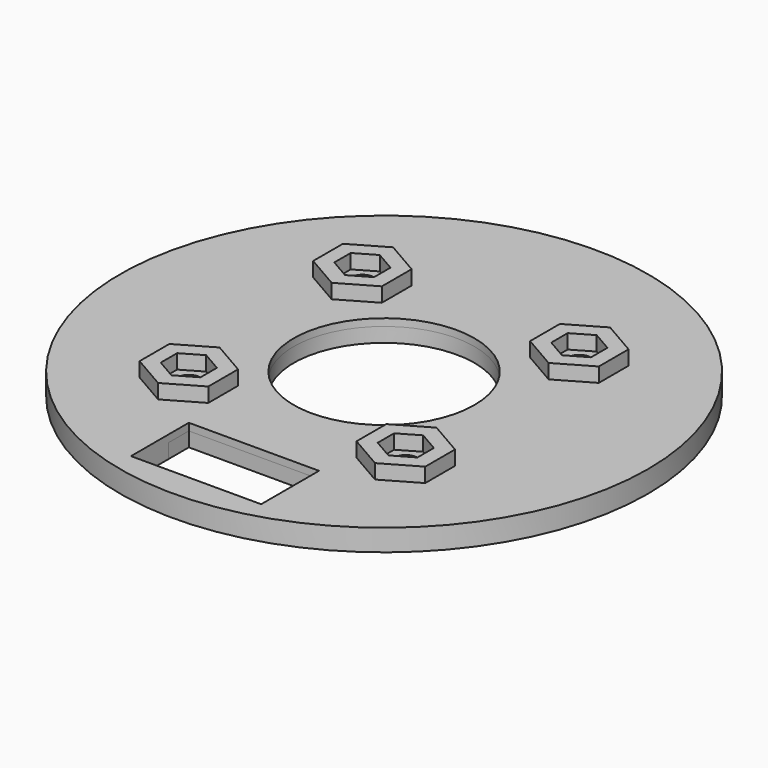
from build123d import *

# Parameters (mm, degrees)
F0_R     = 36.5
F0_R_2   = 12.5
F0_R_3   = 1.6
F1_DEPTH = 3
F2_DEPTH = 5
F3_DEPTH = 2


# Not quite as in the source:
# - a feature names something its author has since deleted; it is built from what else it names


with BuildPart() as f1:
    # F0 (on Top) → F1 (new body)
    with BuildSketch(Plane.XY):
        Circle(F0_R)
        with BuildLine():
            Line((9, -25.9855729204), (9, -32.5))
            Line((9, -32.5), (-9, -32.5))
            Line((-9, -32.5), (-9, -25.9855729204))
            ThreePointArc((-9, -25.9855729204), (-15.9491379077, 22.4025668172), (27.5, 0))
            ThreePointArc((27.5, 0), (22.4025668172, -15.9491379077), (9, -25.9855729204))
        make_face(mode=Mode.SUBTRACT)
        with BuildLine():
            Line((9, -22.5), (9, -25.9855729204))
            ThreePointArc((9, -25.9855729204), (22.4025668172, -15.9491379077), (27.5, 0))
            ThreePointArc((27.5, 0), (-15.9491379077, 22.4025668172), (-9, -25.9855729204))
            Line((-9, -25.9855729204), (-9, -22.5))
            Line((-9, -22.5), (9, -22.5))
        make_face()
        Polygon((-10.25, -12.4280127019), (-10.25, -17.5719872981), (-15, -20.3144010768), (-19.75, -17.5719872981), (-19.75, -12.4280127019), (-15, -9.6855989232), align=None, mode=Mode.SUBTRACT)
        Polygon((15, -20.3144010768), (10.25, -17.5719872981), (10.25, -12.4280127019), (15, -9.6855989232), (19.75, -12.4280127019), (19.75, -17.5719872981), align=None, mode=Mode.SUBTRACT)
        Polygon((-15, 9.6855989232), (-19.75, 12.4280127019), (-19.75, 17.5719872981), (-15, 20.3144010768), (-10.25, 17.5719872981), (-10.25, 12.4280127019), align=None, mode=Mode.SUBTRACT)
        Circle(F0_R_2, mode=Mode.SUBTRACT)
        Polygon((10.25, 12.4280127019), (10.25, 17.5719872981), (15, 20.3144010768), (19.75, 17.5719872981), (19.75, 12.4280127019), (15, 9.6855989232), align=None, mode=Mode.SUBTRACT)
        Polygon((-19.75, 17.5719872981), (-19.75, 12.4280127019), (-15, 9.6855989232), (-10.25, 12.4280127019), (-10.25, 17.5719872981), (-15, 20.3144010768), align=None)
        Polygon((-17.75, 13.5827132403), (-17.75, 16.4172867597), (-15, 18.005), (-12.25, 16.4172867597), (-12.25, 13.5827132403), (-15, 11.995), align=None, mode=Mode.SUBTRACT)
        Polygon((-15, -20.3144010768), (-10.25, -17.5719872981), (-10.25, -12.4280127019), (-15, -9.6855989232), (-19.75, -12.4280127019), (-19.75, -17.5719872981), align=None)
        Polygon((-17.75, -16.4172867597), (-17.75, -13.5827132403), (-15, -11.995), (-12.25, -13.5827132403), (-12.25, -16.4172867597), (-15, -18.005), align=None, mode=Mode.SUBTRACT)
        Polygon((15, 20.3144010768), (10.25, 17.5719872981), (10.25, 12.4280127019), (15, 9.6855989232), (19.75, 12.4280127019), (19.75, 17.5719872981), align=None)
        Polygon((12.25, 13.5827132403), (12.25, 16.4172867597), (15, 18.005), (17.75, 16.4172867597), (17.75, 13.5827132403), (15, 11.995), align=None, mode=Mode.SUBTRACT)
        Polygon((10.25, -12.4280127019), (10.25, -17.5719872981), (15, -20.3144010768), (19.75, -17.5719872981), (19.75, -12.4280127019), (15, -9.6855989232), align=None)
        Polygon((15, -11.995), (17.75, -13.5827132403), (17.75, -16.4172867597), (15, -18.005), (12.25, -16.4172867597), (12.25, -13.5827132403), align=None, mode=Mode.SUBTRACT)
        Polygon((-15, 18.005), (-17.75, 16.4172867597), (-17.75, 13.5827132403), (-15, 11.995), (-12.25, 13.5827132403), (-12.25, 16.4172867597), align=None)
        with Locations((-15, 15)):
            Circle(F0_R_3, mode=Mode.SUBTRACT)
        Polygon((-15, -11.995), (-17.75, -13.5827132403), (-17.75, -16.4172867597), (-15, -18.005), (-12.25, -16.4172867597), (-12.25, -13.5827132403), align=None)
        with Locations((-15, -15)):
            Circle(F0_R_3, mode=Mode.SUBTRACT)
        Polygon((15, 18.005), (12.25, 16.4172867597), (12.25, 13.5827132403), (15, 11.995), (17.75, 13.5827132403), (17.75, 16.4172867597), align=None)
        with Locations((15, 15)):
            Circle(F0_R_3, mode=Mode.SUBTRACT)
        Polygon((17.75, -16.4172867597), (17.75, -13.5827132403), (15, -11.995), (12.25, -13.5827132403), (12.25, -16.4172867597), (15, -18.005), align=None)
        with Locations((15, -15)):
            Circle(F0_R_3, mode=Mode.SUBTRACT)
    extrude(amount=F1_DEPTH)

    # F0 (on Top) → F2 (join)
    with BuildSketch(Plane.XY):
        Polygon((-19.75, 17.5719872981), (-19.75, 12.4280127019), (-15, 9.6855989232), (-10.25, 12.4280127019), (-10.25, 17.5719872981), (-15, 20.3144010768), align=None)
        Polygon((-17.75, 13.5827132403), (-17.75, 16.4172867597), (-15, 18.005), (-12.25, 16.4172867597), (-12.25, 13.5827132403), (-15, 11.995), align=None, mode=Mode.SUBTRACT)
        Polygon((-15, -20.3144010768), (-10.25, -17.5719872981), (-10.25, -12.4280127019), (-15, -9.6855989232), (-19.75, -12.4280127019), (-19.75, -17.5719872981), align=None)
        Polygon((-17.75, -16.4172867597), (-17.75, -13.5827132403), (-15, -11.995), (-12.25, -13.5827132403), (-12.25, -16.4172867597), (-15, -18.005), align=None, mode=Mode.SUBTRACT)
        Polygon((15, 20.3144010768), (10.25, 17.5719872981), (10.25, 12.4280127019), (15, 9.6855989232), (19.75, 12.4280127019), (19.75, 17.5719872981), align=None)
        Polygon((12.25, 13.5827132403), (12.25, 16.4172867597), (15, 18.005), (17.75, 16.4172867597), (17.75, 13.5827132403), (15, 11.995), align=None, mode=Mode.SUBTRACT)
        Polygon((10.25, -12.4280127019), (10.25, -17.5719872981), (15, -20.3144010768), (19.75, -17.5719872981), (19.75, -12.4280127019), (15, -9.6855989232), align=None)
        Polygon((15, -11.995), (17.75, -13.5827132403), (17.75, -16.4172867597), (15, -18.005), (12.25, -16.4172867597), (12.25, -13.5827132403), align=None, mode=Mode.SUBTRACT)
    extrude(amount=F2_DEPTH)


with BuildPart() as f3:
    # F0 (on Top) → F3 (new body)
    with BuildSketch(Plane.XY):
        with BuildLine():
            Line((9, -22.5), (9, -25.9855729204))
            ThreePointArc((9, -25.9855729204), (22.4025668172, -15.9491379077), (27.5, 0))
            ThreePointArc((27.5, 0), (-15.9491379077, 22.4025668172), (-9, -25.9855729204))
            Line((-9, -25.9855729204), (-9, -22.5))
            Line((-9, -22.5), (9, -22.5))
        make_face()
        Polygon((-10.25, -12.4280127019), (-10.25, -17.5719872981), (-15, -20.3144010768), (-19.75, -17.5719872981), (-19.75, -12.4280127019), (-15, -9.6855989232), align=None, mode=Mode.SUBTRACT)
        Polygon((15, -20.3144010768), (10.25, -17.5719872981), (10.25, -12.4280127019), (15, -9.6855989232), (19.75, -12.4280127019), (19.75, -17.5719872981), align=None, mode=Mode.SUBTRACT)
        Polygon((-15, 9.6855989232), (-19.75, 12.4280127019), (-19.75, 17.5719872981), (-15, 20.3144010768), (-10.25, 17.5719872981), (-10.25, 12.4280127019), align=None, mode=Mode.SUBTRACT)
        Circle(F0_R_2, mode=Mode.SUBTRACT)
        Polygon((10.25, 12.4280127019), (10.25, 17.5719872981), (15, 20.3144010768), (19.75, 17.5719872981), (19.75, 12.4280127019), (15, 9.6855989232), align=None, mode=Mode.SUBTRACT)
        Polygon((-19.75, 17.5719872981), (-19.75, 12.4280127019), (-15, 9.6855989232), (-10.25, 12.4280127019), (-10.25, 17.5719872981), (-15, 20.3144010768), align=None)
        Polygon((-17.75, 13.5827132403), (-17.75, 16.4172867597), (-15, 18.005), (-12.25, 16.4172867597), (-12.25, 13.5827132403), (-15, 11.995), align=None, mode=Mode.SUBTRACT)
        Polygon((15, 20.3144010768), (10.25, 17.5719872981), (10.25, 12.4280127019), (15, 9.6855989232), (19.75, 12.4280127019), (19.75, 17.5719872981), align=None)
        Polygon((12.25, 13.5827132403), (12.25, 16.4172867597), (15, 18.005), (17.75, 16.4172867597), (17.75, 13.5827132403), (15, 11.995), align=None, mode=Mode.SUBTRACT)
        Polygon((-15, -20.3144010768), (-10.25, -17.5719872981), (-10.25, -12.4280127019), (-15, -9.6855989232), (-19.75, -12.4280127019), (-19.75, -17.5719872981), align=None)
        Polygon((-17.75, -16.4172867597), (-17.75, -13.5827132403), (-15, -11.995), (-12.25, -13.5827132403), (-12.25, -16.4172867597), (-15, -18.005), align=None, mode=Mode.SUBTRACT)
        Polygon((10.25, -12.4280127019), (10.25, -17.5719872981), (15, -20.3144010768), (19.75, -17.5719872981), (19.75, -12.4280127019), (15, -9.6855989232), align=None)
        Polygon((15, -11.995), (17.75, -13.5827132403), (17.75, -16.4172867597), (15, -18.005), (12.25, -16.4172867597), (12.25, -13.5827132403), align=None, mode=Mode.SUBTRACT)
    extrude(amount=F3_DEPTH)


solid = Compound([f1.part, f3.part])
